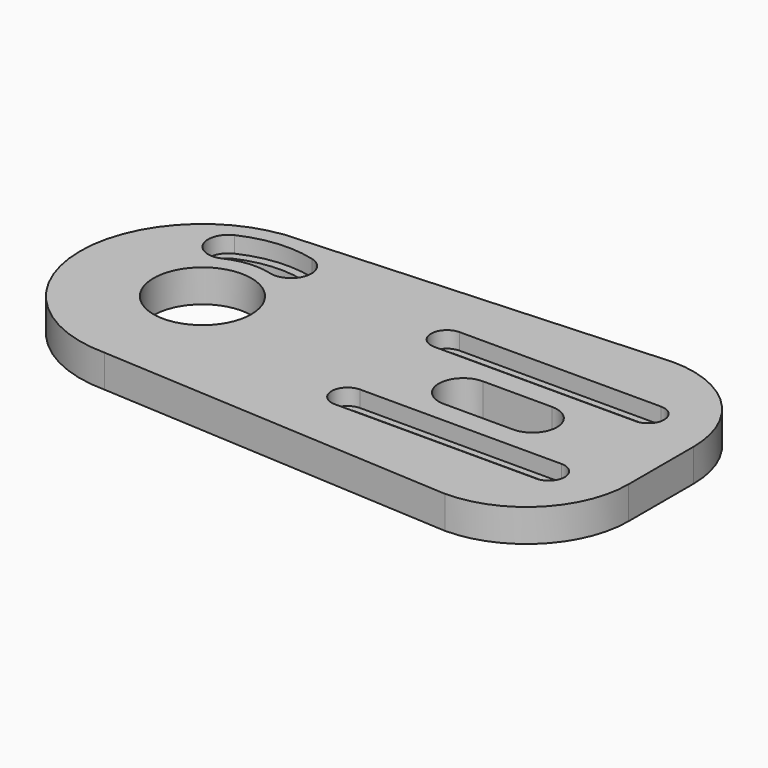
from build123d import *

# Parameters (mm, degrees)
F0_R     = 12
F1_DEPTH = 4
F2_DEPTH = 4


# Not quite as in the source:
# - a feature names something its author has since deleted; it is built from what else it names


with BuildPart() as f1:
    # F0 (on Top) → F1 (new body)
    with BuildSketch(Plane.XY):
        with BuildLine():
            Line((64.1499952853, -10.0000936452), (64.1499952853, 9.9999063548))
            ThreePointArc((64.1499952853, 9.9999063548), (56.8276648149, 27.6775758844), (39.1499952853, 34.9999063548))
            Line((39.1499952853, 34.9999063548), (-48.3500047147, 29.9999063548))
            ThreePointArc((-48.3500047147, 29.9999063548), (-78.3500047147, -9.36452e-05), (-48.3500047147, -30.0000936452))
            Line((-48.3500047147, -30.0000936452), (39.1499952853, -35.0000936452))
            ThreePointArc((39.1499952853, -35.0000936452), (56.8276648149, -27.6777631749), (64.1499952853, -10.0000936452))
        make_face()
        with BuildLine():
            ThreePointArc((-0.5500047147, -19.1500936452), (-4.4500047147, -15.2500936452), (-0.5500047147, -11.3500936452))
            Line((-0.5500047147, -11.3500936452), (24.1499952853, -11.3500936452))
            Line((24.1499952853, -11.3500936452), (48.8499952853, -11.3500936452))
            ThreePointArc((48.8499952853, -11.3500936452), (52.7499952853, -15.2500936452), (48.8499952853, -19.1500936452))
            Line((48.8499952853, -19.1500936452), (24.1499952853, -19.1500936452))
            Line((24.1499952853, -19.1500936452), (-0.5500047147, -19.1500936452))
        make_face(mode=Mode.SUBTRACT)
        with Locations((-48.3500047147, -9.36452e-05)):
            Circle(F0_R, mode=Mode.SUBTRACT)
        with BuildLine():
            ThreePointArc((-55.1419234399, 14.5971608922), (-61.784523832, 17.0211782252), (-59.3605064989, 23.6637786173))
            ThreePointArc((-59.3605064989, 23.6637786173), (-50.6247696004, 26.0005879749), (-41.615965488, 25.2162247953))
            ThreePointArc((-41.615965488, 25.2162247953), (-38.075298972, 19.0954666215), (-44.1960571458, 15.5548001054))
            ThreePointArc((-44.1960571458, 15.5548001054), (-49.753212173, 16.038640994), (-55.1419234399, 14.5971608922))
        make_face(mode=Mode.SUBTRACT)
        with BuildLine():
            Line((24.1499952853, 5.9999063548), (32.6499952853, 5.9999063548))
            ThreePointArc((32.6499952853, 5.9999063548), (38.6499952853, -9.36452e-05), (32.6499952853, -6.0000936452))
            Line((32.6499952853, -6.0000936452), (24.1499952853, -6.0000936452))
            Line((24.1499952853, -6.0000936452), (15.6499952853, -6.0000936452))
            ThreePointArc((15.6499952853, -6.0000936452), (9.6499952853, -9.36452e-05), (15.6499952853, 5.9999063548))
            Line((15.6499952853, 5.9999063548), (24.1499952853, 5.9999063548))
        make_face(mode=Mode.SUBTRACT)
        with BuildLine():
            Line((24.1499952853, 11.3499063548), (-0.5500047147, 11.3499063548))
            ThreePointArc((-0.5500047147, 11.3499063548), (-4.4500047147, 15.2499063548), (-0.5500047147, 19.1499063548))
            Line((-0.5500047147, 19.1499063548), (24.1499952853, 19.1499063548))
            Line((24.1499952853, 19.1499063548), (48.8499952853, 19.1499063548))
            ThreePointArc((48.8499952853, 19.1499063548), (52.7499952853, 15.2499063548), (48.8499952853, 11.3499063548))
            Line((48.8499952853, 11.3499063548), (24.1499952853, 11.3499063548))
        make_face(mode=Mode.SUBTRACT)
        with BuildLine():
            ThreePointArc((-41.615965488, 25.2162247953), (-50.6247696004, 26.0005879749), (-59.3605064989, 23.6637786173))
            ThreePointArc((-59.3605064989, 23.6637786173), (-61.784523832, 17.0211782252), (-55.1419234399, 14.5971608922))
            ThreePointArc((-55.1419234399, 14.5971608922), (-49.753212173, 16.038640994), (-44.1960571458, 15.5548001054))
            ThreePointArc((-44.1960571458, 15.5548001054), (-38.075298972, 19.0954666215), (-41.615965488, 25.2162247953))
        make_face()
        with BuildLine():
            ThreePointArc((-56.0278258823, 16.5011506145), (-59.8805341097, 17.9070806676), (-58.4746040565, 21.7597888951))
            ThreePointArc((-58.4746040565, 21.7597888951), (-50.4417425407, 23.908579109), (-42.1577847361, 23.1873256104))
            ThreePointArc((-42.1577847361, 23.1873256104), (-40.1041981568, 19.6372858696), (-43.6542378976, 17.5836992903))
            ThreePointArc((-43.6542378976, 17.5836992903), (-49.9362392327, 18.13064986), (-56.0278258823, 16.5011506145))
        make_face(mode=Mode.SUBTRACT)
        with BuildLine():
            ThreePointArc((-0.5500047147, 19.1499063548), (-4.4500047147, 15.2499063548), (-0.5500047147, 11.3499063548))
            Line((-0.5500047147, 11.3499063548), (24.1499952853, 11.3499063548))
            Line((24.1499952853, 11.3499063548), (48.8499952853, 11.3499063548))
            ThreePointArc((48.8499952853, 11.3499063548), (52.7499952853, 15.2499063548), (48.8499952853, 19.1499063548))
            Line((48.8499952853, 19.1499063548), (24.1499952853, 19.1499063548))
            Line((24.1499952853, 19.1499063548), (-0.5500047147, 19.1499063548))
        make_face()
        with BuildLine():
            Line((24.1499952853, 13.0499063548), (-0.5500047147, 13.0499063548))
            ThreePointArc((-0.5500047147, 13.0499063548), (-2.7500047147, 15.2499063548), (-0.5500047147, 17.4499063548))
            Line((-0.5500047147, 17.4499063548), (24.1499952853, 17.4499063548))
            Line((24.1499952853, 17.4499063548), (48.8499952853, 17.4499063548))
            ThreePointArc((48.8499952853, 17.4499063548), (51.0499952853, 15.2499063548), (48.8499952853, 13.0499063548))
            Line((48.8499952853, 13.0499063548), (24.1499952853, 13.0499063548))
        make_face(mode=Mode.SUBTRACT)
        with BuildLine():
            Line((24.1499952853, -11.3500936452), (-0.5500047147, -11.3500936452))
            ThreePointArc((-0.5500047147, -11.3500936452), (-4.4500047147, -15.2500936452), (-0.5500047147, -19.1500936452))
            Line((-0.5500047147, -19.1500936452), (24.1499952853, -19.1500936452))
            Line((24.1499952853, -19.1500936452), (48.8499952853, -19.1500936452))
            ThreePointArc((48.8499952853, -19.1500936452), (52.7499952853, -15.2500936452), (48.8499952853, -11.3500936452))
            Line((48.8499952853, -11.3500936452), (24.1499952853, -11.3500936452))
        make_face()
        with BuildLine():
            ThreePointArc((-0.5500047147, -17.4500936452), (-2.7500047147, -15.2500936452), (-0.5500047147, -13.0500936452))
            Line((-0.5500047147, -13.0500936452), (24.1499952853, -13.0500936452))
            Line((24.1499952853, -13.0500936452), (48.8499952853, -13.0500936452))
            ThreePointArc((48.8499952853, -13.0500936452), (51.0499952853, -15.2500936452), (48.8499952853, -17.4500936452))
            Line((48.8499952853, -17.4500936452), (24.1499952853, -17.4500936452))
            Line((24.1499952853, -17.4500936452), (-0.5500047147, -17.4500936452))
        make_face(mode=Mode.SUBTRACT)
    extrude(amount=-F1_DEPTH)

    # F0 (on Top) → F2 (join)
    with BuildSketch(Plane.XY):
        with BuildLine():
            Line((64.1499952853, -10.0000936452), (64.1499952853, 9.9999063548))
            ThreePointArc((64.1499952853, 9.9999063548), (56.8276648149, 27.6775758844), (39.1499952853, 34.9999063548))
            Line((39.1499952853, 34.9999063548), (-48.3500047147, 29.9999063548))
            ThreePointArc((-48.3500047147, 29.9999063548), (-78.3500047147, -9.36452e-05), (-48.3500047147, -30.0000936452))
            Line((-48.3500047147, -30.0000936452), (39.1499952853, -35.0000936452))
            ThreePointArc((39.1499952853, -35.0000936452), (56.8276648149, -27.6777631749), (64.1499952853, -10.0000936452))
        make_face()
        with BuildLine():
            ThreePointArc((-0.5500047147, -19.1500936452), (-4.4500047147, -15.2500936452), (-0.5500047147, -11.3500936452))
            Line((-0.5500047147, -11.3500936452), (24.1499952853, -11.3500936452))
            Line((24.1499952853, -11.3500936452), (48.8499952853, -11.3500936452))
            ThreePointArc((48.8499952853, -11.3500936452), (52.7499952853, -15.2500936452), (48.8499952853, -19.1500936452))
            Line((48.8499952853, -19.1500936452), (24.1499952853, -19.1500936452))
            Line((24.1499952853, -19.1500936452), (-0.5500047147, -19.1500936452))
        make_face(mode=Mode.SUBTRACT)
        with Locations((-48.3500047147, -9.36452e-05)):
            Circle(F0_R, mode=Mode.SUBTRACT)
        with BuildLine():
            ThreePointArc((-55.1419234399, 14.5971608922), (-61.784523832, 17.0211782252), (-59.3605064989, 23.6637786173))
            ThreePointArc((-59.3605064989, 23.6637786173), (-50.6247696004, 26.0005879749), (-41.615965488, 25.2162247953))
            ThreePointArc((-41.615965488, 25.2162247953), (-38.075298972, 19.0954666215), (-44.1960571458, 15.5548001054))
            ThreePointArc((-44.1960571458, 15.5548001054), (-49.753212173, 16.038640994), (-55.1419234399, 14.5971608922))
        make_face(mode=Mode.SUBTRACT)
        with BuildLine():
            Line((24.1499952853, 5.9999063548), (32.6499952853, 5.9999063548))
            ThreePointArc((32.6499952853, 5.9999063548), (38.6499952853, -9.36452e-05), (32.6499952853, -6.0000936452))
            Line((32.6499952853, -6.0000936452), (24.1499952853, -6.0000936452))
            Line((24.1499952853, -6.0000936452), (15.6499952853, -6.0000936452))
            ThreePointArc((15.6499952853, -6.0000936452), (9.6499952853, -9.36452e-05), (15.6499952853, 5.9999063548))
            Line((15.6499952853, 5.9999063548), (24.1499952853, 5.9999063548))
        make_face(mode=Mode.SUBTRACT)
        with BuildLine():
            Line((24.1499952853, 11.3499063548), (-0.5500047147, 11.3499063548))
            ThreePointArc((-0.5500047147, 11.3499063548), (-4.4500047147, 15.2499063548), (-0.5500047147, 19.1499063548))
            Line((-0.5500047147, 19.1499063548), (24.1499952853, 19.1499063548))
            Line((24.1499952853, 19.1499063548), (48.8499952853, 19.1499063548))
            ThreePointArc((48.8499952853, 19.1499063548), (52.7499952853, 15.2499063548), (48.8499952853, 11.3499063548))
            Line((48.8499952853, 11.3499063548), (24.1499952853, 11.3499063548))
        make_face(mode=Mode.SUBTRACT)
    extrude(amount=F2_DEPTH)


solid = f1.part
